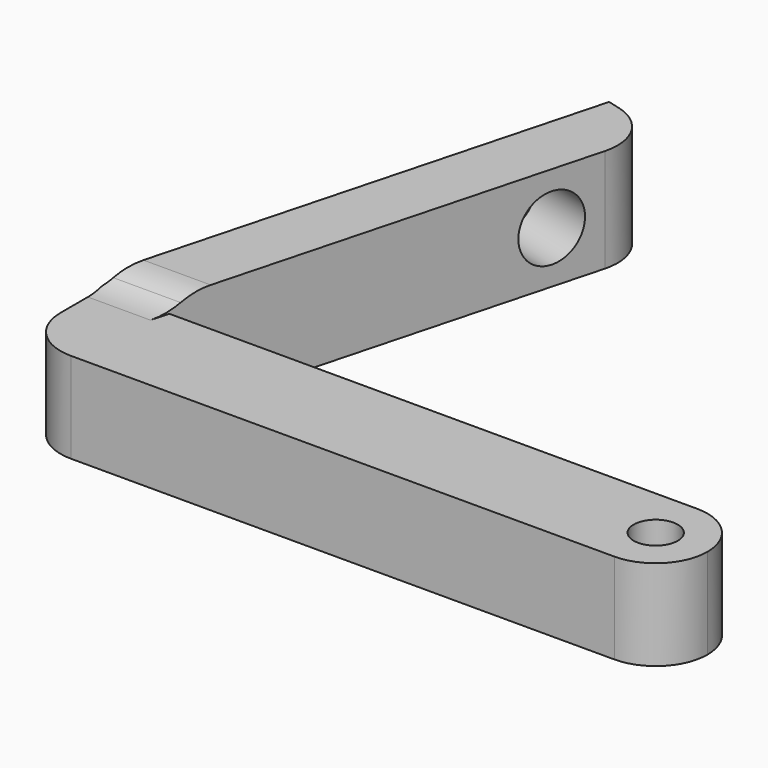
from build123d import *

# Parameters (mm, degrees)
F1_DEPTH    = 7
F2_DEPTH    = 8
F3_R        = 3.99999
F4_T1_DEPTH = 20.2030500331
F5_R        = 5
F6_R        = 2.5
F7_DEPTH    = 10
F6_R_2      = 3
F8_DEPTH    = 4.6
F9_R        = 1.7
F10_DEPTH   = 7.001


# Not quite as in the source:
# - a fillet or chamfer that OpenCascade refuses, or shapes differently, is made with other operations: its cross-section is extruded or revolved along the edge and cut away or added
# - a fillet or chamfer is up to 0.001 mm smaller than in the source, because OpenCascade refuses the exact size


with BuildPart() as f1:
    # F0 (on Top) → F1 (new body)
    with BuildSketch(Plane.XY):
        Polygon((-25, -4), (25, -4), (25, 4), (-19.7969499669, 4), (-25, 4), align=None)
    extrude(amount=F1_DEPTH)

    # F0 (on Top) → F2 (join)
    with BuildSketch(Plane.XY):
        Polygon((-15.1648762861, 40.705181399), (-25, 4), (-19.7969499669, 4), (-10.3103645166, 39.4044188907), align=None)
    extrude(amount=F2_DEPTH)

    # F3 (radius 4 in the source; OpenCascade refuses exactly that, so slightly less here)
    f3_edges = [f1.edges().sort_by_distance(p)[0] for p in [
        (25, 4, 3.5),
        (25, -4, 3.5),
        (-25, -4, 3.5),
        (-10.310365, 39.404419, 4),
    ]]
    fillet(f3_edges, radius=F3_R)

    # F4: fillet of radius 5 on 1 edges, made by hand

    # F4_s2 → F4_t1 (cut)
    with BuildSketch(Plane.YZ.offset(-32.5)):
        with BuildLine():
            ThreePointArc((4, 7), (5.4188611699, 7.7434164903), (7, 8))
            Line((7, 8), (4, 8))
            Line((4, 8), (4, 7))
        make_face()
    extrude(amount=F4_T1_DEPTH, mode=Mode.SUBTRACT)

    # F5
    f5_edges = [f1.edges().sort_by_distance(p)[0] for p in [
        (-22.398475, 4, 7),
    ]]
    fillet(f5_edges, radius=F5_R)

    # F6 (on face) → F7 (cut)
    with BuildSketch(Plane(origin=(-24.3253175473, 6.5179491924, 0), x_dir=(-0.2588190451, -0.9659258263, 0), z_dir=(-0.9659258263, 0.2588190451, 0))):
        with Locations((-27.3932271776, 4)):
            Circle(F6_R)
    extrude(amount=-F7_DEPTH, mode=Mode.SUBTRACT)

    # F6 (on face) → F8 (cut)
    with BuildSketch(Plane(origin=(-24.3253175473, 6.5179491924, 0), x_dir=(-0.2588190451, -0.9659258263, 0), z_dir=(-0.9659258263, 0.2588190451, 0))):
        with Locations((-8.3932271776, 4)):
            Circle(F6_R_2)
    extrude(amount=-F8_DEPTH, mode=Mode.SUBTRACT)

    # F9 (on face) → F10 (cut, through all)
    with BuildSketch(Plane.XY.offset(7)):
        with Locations((21, 0)):
            Circle(F9_R)
    extrude(amount=-F10_DEPTH, mode=Mode.SUBTRACT)


solid = f1.part
